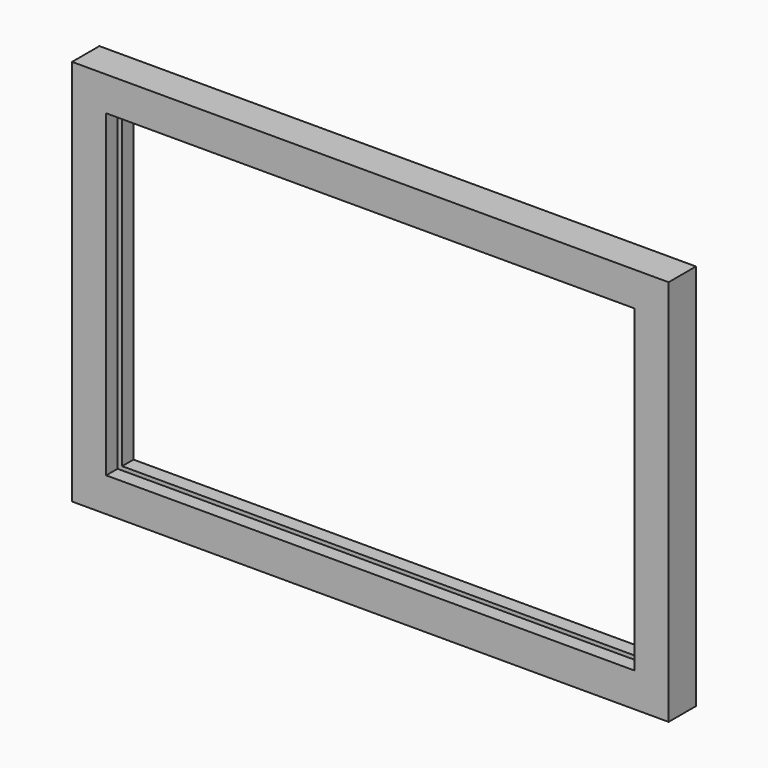
from build123d import *

# Parameters (mm, degrees)
F0_W          = 332.74
F0_H          = 215.9
F0_W_2        = 294.64
F0_H_2        = 177.8
F1_DEPTH      = 9.525
F1_DEPTH_BACK = 9.525
F2_W          = 307.34
F2_H          = 190.5
F3_DEPTH      = 0.0625
F3_DEPTH_BACK = 1.6002


# Not quite as in the source:
# - a pattern or mirror of a feature is missing from the dataset's text; its kind, count and spacing are read off the source's solid


with BuildPart() as f1:
    # F0 (on Front) → F1 (new body, two sides)
    with BuildSketch(Plane.XZ) as f1_sk:
        Rectangle(F0_W, F0_H)
        Rectangle(F0_W_2, F0_H_2, mode=Mode.SUBTRACT)
    extrude(amount=F1_DEPTH)
    extrude(f1_sk.sketch, amount=-F1_DEPTH_BACK)

    # F2 (on Front) → F3 (cut, two sides)
    with BuildSketch(Plane.XZ) as f3_sk:
        Rectangle(F2_W, F2_H)
    f3 = extrude(amount=-F3_DEPTH, mode=Mode.SUBTRACT) + extrude(f3_sk.sketch, amount=F3_DEPTH_BACK, mode=Mode.SUBTRACT)

    # F3_copies: F3 across plane
    add(f3.mirror(Plane.ZX.offset(-0.00635)), mode=Mode.SUBTRACT)


solid = f1.part
